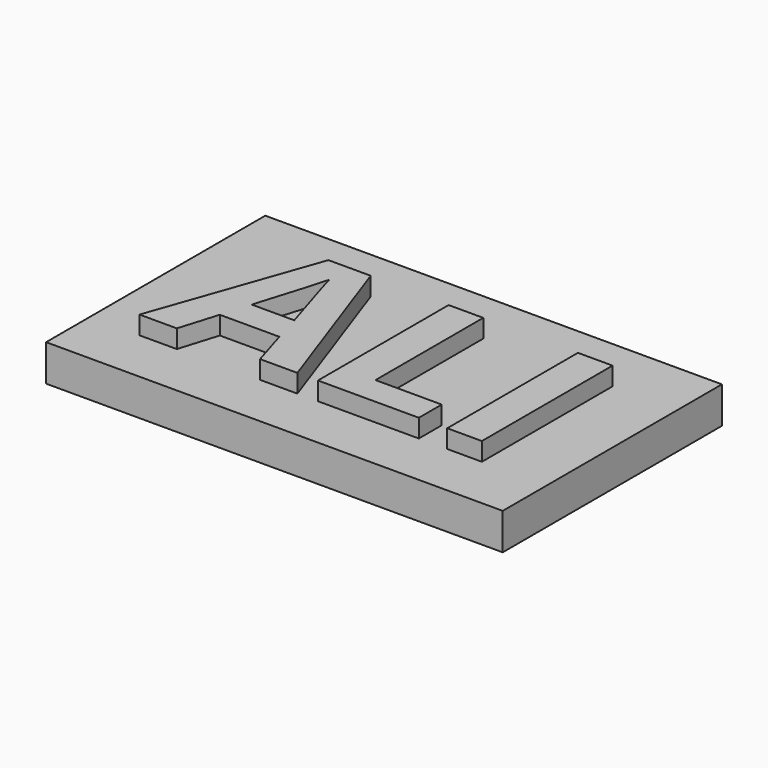
from build123d import *

# Parameters (mm, degrees)
F0_W         = 50
F0_H         = 30
F1_DEPTH     = 4
F2_TEXT_SIZE = 25.0548495719
F3_DEPTH     = 2


# Not quite as in the source:
# - Text() gives the source's letters only with a copy of the font that has no kerning and outlines rounded to 1/6400 em; it was checked with that copy


with BuildPart() as f1:
    # F0 (on Top) → F1 (new body)
    with BuildSketch(Plane.XY):
        Rectangle(F0_W, F0_H)
    extrude(amount=F1_DEPTH)

    # F2 (on face) → F3 (join)
    with BuildSketch(Plane.XY.offset(4)):
        with Locations((-19.5564845369, -9.0197458459)):
            Text('ALI', F2_TEXT_SIZE, font='Open Sans', font_style=FontStyle.BOLD, text_align=(TextAlign.LEFT, TextAlign.BOTTOM))
    extrude(amount=F3_DEPTH)


solid = f1.part
